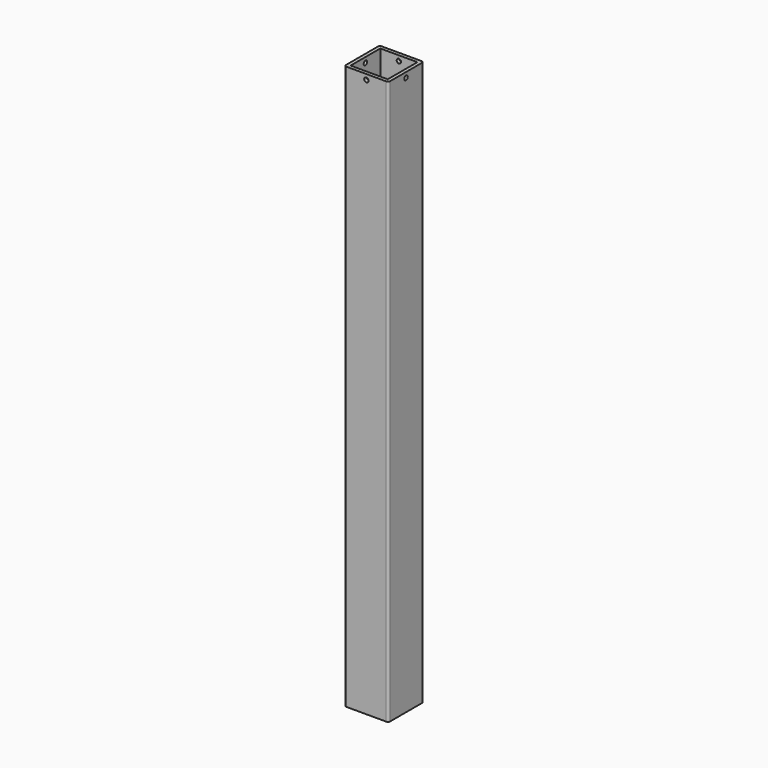
from build123d import *

# Parameters (mm, degrees)
F0_W            = 42.8
F0_H            = 42.8
F1_DEPTH        = 650
F3_D            = 5
F3_DEPTH        = 15
F3_TIP          = 1.5021515476
F3_COPIES_COUNT = 4


# Not quite as in the source:
# - a pattern or mirror of a feature is missing from the dataset's text; its kind, count and spacing are read off the source's solid


with BuildPart() as f1:
    # F0 (on Top) → F1 (new body)
    with BuildSketch(Plane.XY):
        with BuildLine():
            Line((-0.3117055804, 27.0466537178), (-46.1117055804, 27.0466537178))
            ThreePointArc((-46.1117055804, 27.0466537178), (-47.8794725333, 26.3144206707), (-48.6117055804, 24.5466537178))
            Line((-48.6117055804, 24.5466537178), (-48.6117055804, -21.2533462822))
            ThreePointArc((-48.6117055804, -21.2533462822), (-47.8794725333, -23.0211132352), (-46.1117055804, -23.7533462822))
            Line((-46.1117055804, -23.7533462822), (-0.3117055804, -23.7533462822))
            ThreePointArc((-0.3117055804, -23.7533462822), (1.4560613726, -23.0211132352), (2.1882944196, -21.2533462822))
            Line((2.1882944196, -21.2533462822), (2.1882944196, 24.5466537178))
            ThreePointArc((2.1882944196, 24.5466537178), (1.4560613726, 26.3144206707), (-0.3117055804, 27.0466537178))
        make_face()
        with Locations((-23.2117055804, 1.6466537178)):
            Rectangle(F0_W, F0_H, mode=Mode.SUBTRACT)
    extrude(amount=F1_DEPTH)

    # F3
    with Locations(Plane.XZ.offset(23.7533462822)):
        with Locations((-23.2117055804, 644.05)):
            f3 = Hole(F3_D / 2, depth=F3_DEPTH)
            with Locations((0, 0, -(F3_DEPTH + F3_TIP / 2))):  # 118° drill point
                Cone(0, F3_D / 2, F3_TIP, mode=Mode.SUBTRACT)

    # F3_copies: F3 ×4 about axis
    f3_copies_axis = Axis((-23.211706, 1.646654, 0), (0, 0, 1))
    for i in range(1, F3_COPIES_COUNT):
        add(f3.rotate(f3_copies_axis, i * 360 / F3_COPIES_COUNT), mode=Mode.SUBTRACT)


solid = f1.part
